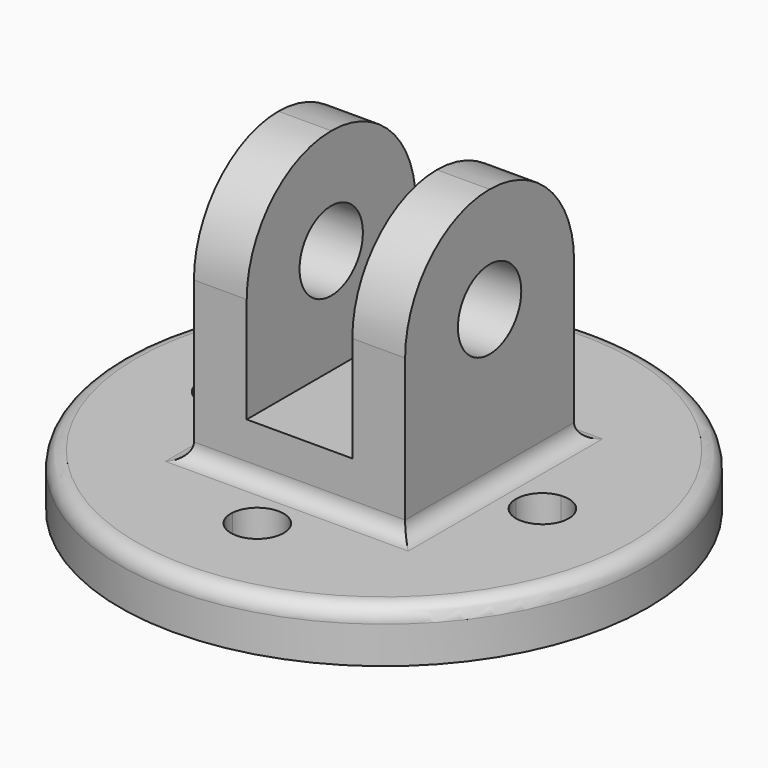
from build123d import *

# Parameters (mm, degrees)
F0_R     = 63.5
F1_DEPTH = 12.7
F3_DEPTH = 63.5
F4_W     = 25.4
F4_H     = 50.8
F5_DEPTH = 50.8
F7_DEPTH = 127
F8_R     = 25.39999
F9_R     = 3.81


# Not quite as in the source:
# - a fillet or chamfer is up to 0.001 mm smaller than in the source, because OpenCascade refuses the exact size


with BuildPart() as f1:
    # F0 (on Top) → F1 (new body)
    with BuildSketch(Plane.XY):
        Circle(F0_R)
        with BuildLine():
            ThreePointArc((6.3279129766, -37.5708333333), (6.3444758413, -37.835186293), (6.35, -38.1))
            ThreePointArc((6.35, -38.1), (-0.264813707, -44.4444758413), (-6.3279129766, -37.5708333333))
            ThreePointArc((-6.3279129766, -37.5708333333), (0, -31.75), (6.3279129766, -37.5708333333))
        make_face(mode=Mode.SUBTRACT)
        with BuildLine():
            ThreePointArc((-37.5708333333, 6.3279129766), (-33.4265265416, 4.2989703225), (-31.75, 0))
            ThreePointArc((-31.75, 0), (-33.4265265416, -4.2989703225), (-37.5708333333, -6.3279129766))
            ThreePointArc((-37.5708333333, -6.3279129766), (-44.45, 0), (-37.5708333333, 6.3279129766))
        make_face(mode=Mode.SUBTRACT)
        with BuildLine():
            ThreePointArc((37.5708333333, -6.3279129766), (33.4265265416, -4.2989703225), (31.75, 0))
            ThreePointArc((31.75, 0), (33.4265265416, 4.2989703225), (37.5708333333, 6.3279129766))
            ThreePointArc((37.5708333333, 6.3279129766), (42.3989703225, 4.6734734584), (44.45, 0))
            ThreePointArc((44.45, 0), (42.3989703225, -4.6734734584), (37.5708333333, -6.3279129766))
        make_face(mode=Mode.SUBTRACT)
        with BuildLine():
            ThreePointArc((6.35, 38.1), (6.3444758413, 37.835186293), (6.3279129766, 37.5708333333))
            ThreePointArc((6.3279129766, 37.5708333333), (4.2989703225, 33.4265265416), (0, 31.75))
            ThreePointArc((0, 31.75), (-4.2989703225, 33.4265265416), (-6.3279129766, 37.5708333333))
            ThreePointArc((-6.3279129766, 37.5708333333), (-0.264813707, 44.4444758413), (6.35, 38.1))
        make_face(mode=Mode.SUBTRACT)
    extrude(amount=F1_DEPTH)

    # F2 (on face) → F3 (join)
    with BuildSketch(Plane.XY.offset(12.7)):
        Polygon((25.4, 25.4), (0, 25.4), (-25.4, 25.4), (-25.4, -25.4), (25.4, -25.4), align=None)
    extrude(amount=F3_DEPTH)

    # F4 (on face) → F5 (cut)
    with BuildSketch(Plane.XZ.offset(25.4)):
        with Locations((0, 50.8)):
            Rectangle(F4_W, F4_H)
    extrude(amount=-F5_DEPTH, mode=Mode.SUBTRACT)

    # F6 (on face) → F7 (cut)
    with BuildSketch(Plane.YZ.offset(25.4)):
        with BuildLine():
            ThreePointArc((9.525, 50.8), (6.7351920908, 57.5351920908), (0, 60.325))
            Line((0, 60.325), (0, 50.8))
            Line((0, 50.8), (0, 41.275))
            ThreePointArc((0, 41.275), (6.7351920908, 44.0648079092), (9.525, 50.8))
        make_face()
        with BuildLine():
            Line((0, 50.8), (0, 60.325))
            ThreePointArc((0, 60.325), (-9.525, 50.8), (0, 41.275))
            Line((0, 41.275), (0, 50.8))
        make_face()
    extrude(amount=-F7_DEPTH, mode=Mode.SUBTRACT)

    # F8 (radius 25.4 in the source; OpenCascade refuses exactly that, so slightly less here)
    f8_edges = [f1.edges().sort_by_distance(p)[0] for p in [
        (19.05, -25.4, 76.2),
        (19.05, 25.4, 76.2),
        (-19.05, -25.4, 76.2),
        (-19.05, 25.4, 76.2),
    ]]
    fillet(f8_edges, radius=F8_R)

    # F9
    f9_edges = [f1.edges().sort_by_distance(p)[0] for p in [
        (-63.5, 0, 12.7),
        (25.4, 0, 12.7),
        (0, -25.4, 12.7),
        (0, 25.4, 12.7),
        (-25.4, 0, 12.7),
    ]]
    fillet(f9_edges, radius=F9_R)


solid = f1.part
